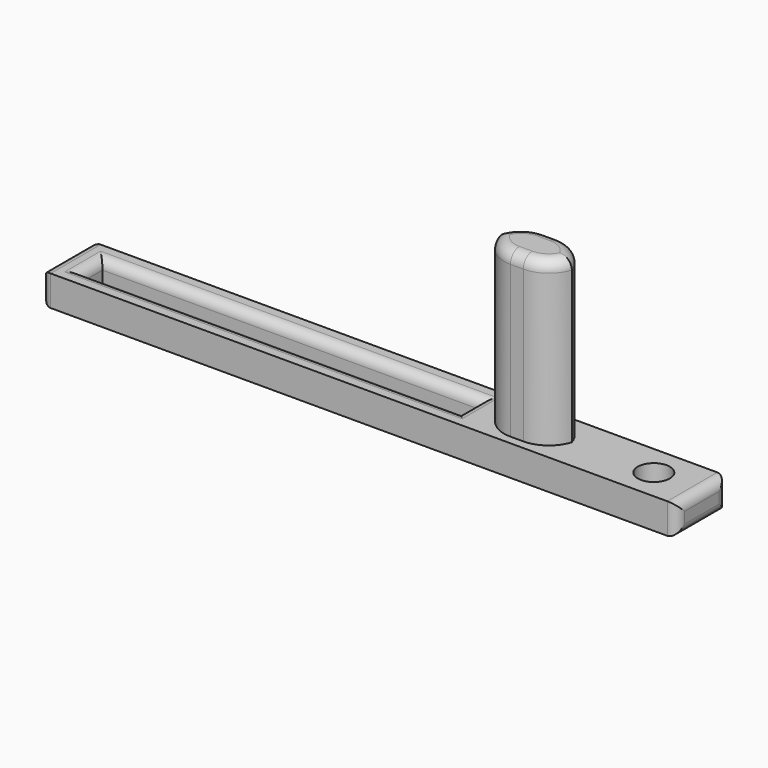
from build123d import *

# Parameters (mm, degrees)
F0_W        = 99.15
F0_H        = 9.75
F1_DEPTH    = 4.75
F2_R        = 2.5
F3_DEPTH    = 4.751
F4_W        = 12
F4_H        = 7
F5_DEPTH    = 25.4
F6_T1_DEPTH = 37.9
F7_R        = 1.5
F8_R        = 1.75
F9_W        = 59
F9_H        = 4
F10_DEPTH   = 25
F11_R       = 1.5


# Not quite as in the source:
# - a fillet or chamfer that OpenCascade refuses, or shapes differently, is made with other operations: its cross-section is extruded or revolved along the edge and cut away or added


with BuildPart() as f1:
    # F0 (on Top) → F1 (new body)
    with BuildSketch(Plane.XY):
        Rectangle(F0_W, F0_H)
    extrude(amount=F1_DEPTH)

    # F2 (on face) → F3 (cut, through all)
    with BuildSketch(Plane.XY.offset(4.75)):
        with Locations((42.075, 0)):
            Circle(F2_R)
    extrude(amount=-F3_DEPTH, mode=Mode.SUBTRACT)

    # F4 (on face) → F5 (join)
    with BuildSketch(Plane.XY.offset(4.75)):
        with Locations((23.525, 0)):
            Rectangle(F4_W, F4_H)
    extrude(amount=F5_DEPTH)

    # F6: fillet of radius 5 on 4 edges, made by hand

    # F6_s2 → F6_t1 (cut)
    with BuildSketch(Plane.XY.offset(4.75)):
        with BuildLine():
            ThreePointArc((22.525, 3.5), (18.9894660941, 2.0355339059), (17.525, -1.5))
            Line((17.525, -1.5), (17.525, 3.5))
            Line((17.525, 3.5), (22.525, 3.5))
        make_face()
        with BuildLine():
            ThreePointArc((17.525, 1.5), (18.9894660941, -2.0355339059), (22.525, -3.5))
            Line((22.525, -3.5), (17.525, -3.5))
            Line((17.525, -3.5), (17.525, 1.5))
        make_face()
        with BuildLine():
            ThreePointArc((29.525, -1.5), (28.0605339059, 2.0355339059), (24.525, 3.5))
            Line((24.525, 3.5), (29.525, 3.5))
            Line((29.525, 3.5), (29.525, -1.5))
        make_face()
        with BuildLine():
            ThreePointArc((29.525, 1.5), (28.0605339059, -2.0355339059), (24.525, -3.5))
            Line((24.525, -3.5), (29.525, -3.5))
            Line((29.525, -3.5), (29.525, 1.5))
        make_face()
    extrude(amount=F6_T1_DEPTH, mode=Mode.SUBTRACT)

    # F7
    f7_edges = [f1.edges().sort_by_distance(p)[0] for p in [
        (-49.575, 4.875, 2.375),
        (-49.575, -4.875, 2.375),
        (-49.575, 0, 0),
        (-49.575, 0, 4.75),
        (49.575, -4.875, 2.375),
        (49.575, 4.875, 2.375),
        (49.575, 0, 0),
        (49.575, 0, 4.75),
    ]]
    fillet(f7_edges, radius=F7_R)

    # F8
    f8_edges = [f1.edges().sort_by_distance(p)[0] for p in [
        (23.525, -3.5, 30.15),
        (19.56696, -2.531129, 30.15),
        (19.56696, 2.531129, 30.15),
        (23.525, 3.5, 30.15),
        (27.48304, 2.531129, 30.15),
        (27.48304, -2.531129, 30.15),
    ]]
    fillet(f8_edges, radius=F8_R)

    # F9 (on face) → F10 (cut)
    with BuildSketch(Plane.XY.offset(4.75)):
        with Locations((-16, 0)):
            Rectangle(F9_W, F9_H)
    extrude(amount=-F10_DEPTH, mode=Mode.SUBTRACT)

    # F11
    f11_edges = [f1.edges().sort_by_distance(p)[0] for p in [
        (-16, 2, 4.75),
        (-45.5, 0, 4.75),
        (-16, -2, 4.75),
        (13.5, 0, 4.75),
        (13.5, 0, 0),
        (-16, 2, 0),
        (-16, -2, 0),
        (-45.5, 0, 0),
    ]]
    fillet(f11_edges, radius=F11_R)


solid = f1.part
